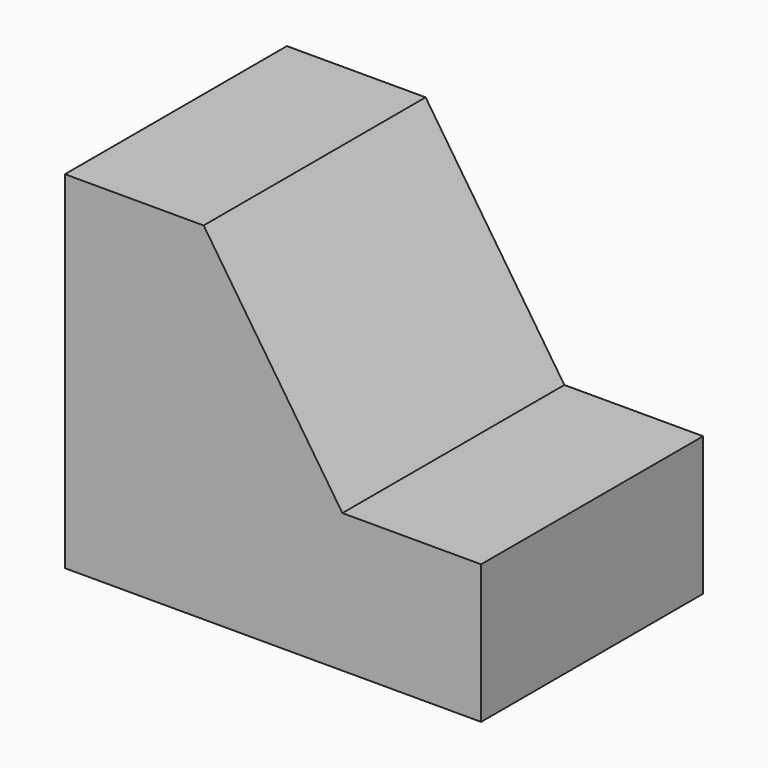
from build123d import *

# Parameters (mm, degrees)
F1_DEPTH = 25.4
F3_DEPTH = 25.4


# Not quite as in the source:
# - a feature names something its author has since deleted; it is built from what else it names


with BuildPart() as f1:
    # F0 (on Front) → F1 (new body)
    with BuildSketch(Plane.XZ):
        Polygon((38.1, 31.75), (12.7, 31.75), (25.4, 12.7), (38.1, 12.7), align=None)
        Polygon((0, 31.75), (0, 0), (25.4, 0), (38.1, 0), (38.1, 12.7), (25.4, 12.7), (12.7, 31.75), align=None)
    extrude(amount=F1_DEPTH)

    # F0 (on Front) → F3 (cut)
    with BuildSketch(Plane.XZ):
        Polygon((38.1, 31.75), (12.7, 31.75), (25.4, 12.7), (38.1, 12.7), align=None)
    extrude(amount=F3_DEPTH, mode=Mode.SUBTRACT)


solid = f1.part
